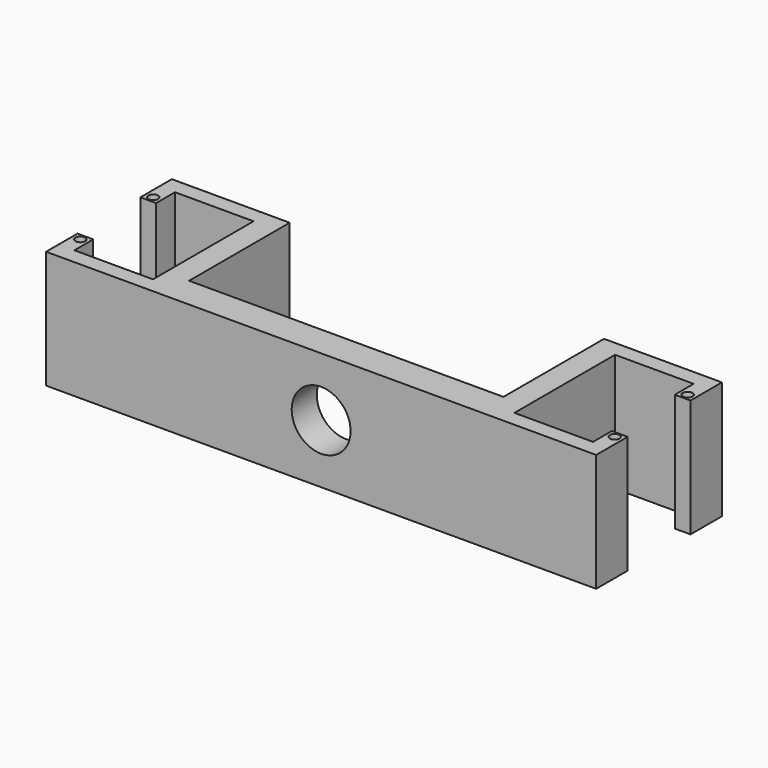
from build123d import *

# Parameters (mm, degrees)
F0_R     = 0.396875
F0_W     = 25.4
F0_H     = 2.54
F1_DEPTH = 4.7625
F2_R     = 2.38125
F3_DEPTH = 5.969


# Not quite as in the source:
# - a length typed as a fraction of an inch, garbled in the dataset ("3 / 203.2 mm" for 3/8 in), is restored
# - a feature names something its author has since deleted; it is built from what else it names


with BuildPart() as f1:
    # F0 (on Top) → F1 (new body, symmetric)
    with BuildSketch(Plane.XY):
        Polygon((-12.7, 11.43), (-22.225, 11.43), (-22.225, 8.255), (-20.955, 8.255), (-20.955, 10.16), (-14.605, 10.16), (-14.605, 0), (-20.955, 0), (-20.955, 1.905), (-22.225, 1.905), (-22.225, -1.27), (-12.7, -1.27), (-12.7, 1.27), align=None)
        with Locations((-21.59, 1.397)):
            Circle(F0_R, mode=Mode.SUBTRACT)
        with Locations((-21.59, 8.763)):
            Circle(F0_R, mode=Mode.SUBTRACT)
        Rectangle(F0_W, F0_H)
        Polygon((12.7, 11.43), (12.7, 1.27), (12.7, -1.27), (22.225, -1.27), (22.225, 1.905), (20.955, 1.905), (20.955, 0), (14.605, 0), (14.605, 10.16), (20.955, 10.16), (20.955, 8.255), (22.225, 8.255), (22.225, 11.43), align=None)
        with Locations((21.59, 1.397)):
            Circle(F0_R, mode=Mode.SUBTRACT)
        with Locations((21.59, 8.763)):
            Circle(F0_R, mode=Mode.SUBTRACT)
    extrude(amount=F1_DEPTH, both=True)

    # F2 (on face) → F3 (cut)
    with BuildSketch(Plane(origin=(0, 1.27, 0), x_dir=(-1, 0, 0), z_dir=(0, 1, 0))):
        Circle(F2_R)
    extrude(amount=-F3_DEPTH, mode=Mode.SUBTRACT)


solid = f1.part
